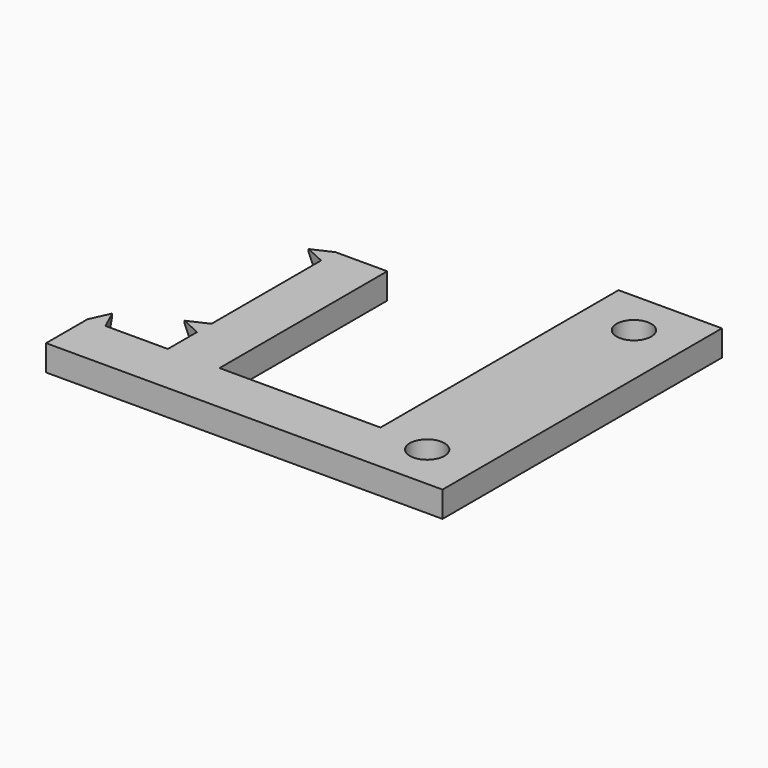
from build123d import *

# Parameters (mm, degrees)
F0_R     = 3.350006
F1_DEPTH = 5
F3_DEPTH = 40.5559613398
F5_DEPTH = 15.5559613398


# Not quite as in the source:
# - a feature names something its author has since deleted; it is built from what else it names


with BuildPart() as f1:
    # F0 (on Top) → F1 (new body)
    with BuildSketch(Plane.XY):
        Polygon((0, 10), (3.4919226796, 10), (1.7459613398, 13.81), align=None)
        Polygon((15.5559613398, 18.81), (15.5559613398, 20.5559613398), (11.7459613398, 18.81), align=None)
        Polygon((15.5559613398, 47.0640386602), (15.5559613398, 50.5559613398), (11.7459613398, 48.81), align=None)
        Polygon((25.5559613398, 50.5559613398), (15.5559613398, 50.5559613398), (15.5559613398, 47.0640386602), (15.5559613398, 20.5559613398), (15.5559613398, 18.81), (15.5559613398, 17.0640386602), (15.5559613398, 10), (3.4919226796, 10), (0, 10), (0, 0), (76.6976781032, 0), (76.6976781032, 67.5584669805), (56.6976781032, 67.5584669805), (56.6976781032, 10), (25.5559613398, 10), align=None)
        with Locations((66.6976781032, 8.7792334903)):
            Circle(F0_R, mode=Mode.SUBTRACT)
        with Locations((66.6976781032, 58.7792334903)):
            Circle(F0_R, mode=Mode.SUBTRACT)
        Polygon((15.5559613398, 17.0640386602), (15.5559613398, 18.81), (11.7459613398, 18.81), align=None)
    extrude(amount=F1_DEPTH)

    # F2 (on face) → F3 (cut, through all)
    with BuildSketch(Plane(origin=(0, 50.5559613398, 0), x_dir=(-1, 0, 0), z_dir=(0, 1, 0))):
        Polygon((-11.7459613398, 4.5), (-15.5559613398, 0), (-11.7459613398, 0), align=None)
    extrude(amount=-F3_DEPTH, mode=Mode.SUBTRACT)

    # F4 (on face) → F5 (cut, through all)
    with BuildSketch(Plane(origin=(0, 0, 0), x_dir=(0, -1, 0), z_dir=(-1, 0, 0))):
        Polygon((-13.81, 0), (-10, 0), (-13.81, 4.5), align=None)
    extrude(amount=-F5_DEPTH, mode=Mode.SUBTRACT)


solid = f1.part
